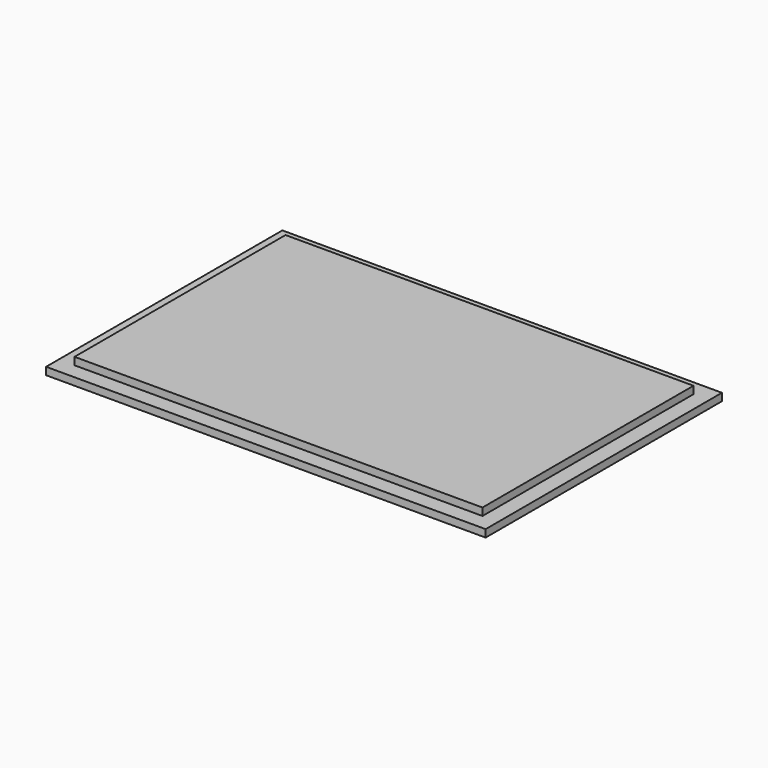
from build123d import *

# Parameters (mm, degrees)
F2_DEPTH = 105.9625
F3_W     = 176.60625
F3_H     = 3
F4_DEPTH = 6.35
F5_W     = 176.60625
F5_H     = 3
F6_DEPTH = 6.35


# Not quite as in the source:
# - a length typed as a fraction of an inch, garbled in the dataset ("3 / 203.2 mm" for 3/8 in), is restored


with BuildPart() as f2:
    # F1 (on Front) → F2 (new body)
    with BuildSketch(Plane.XZ):
        Polygon((-42.2606132925, -1.7798869123), (-42.2606132925, -4.7798869123), (134.3456367075, -4.7798869123), (134.3456367075, -1.7798869123), (127.9956367075, -1.7798869123), (127.9956367075, 1.2201130877), (-35.9106132925, 1.2201130877), (-35.9106132925, -1.7798869123), align=None)
    extrude(amount=F2_DEPTH)

    # F3 (on face) → F4 (join)
    with BuildSketch(Plane.XZ.offset(105.9625)):
        with Locations((46.0425117075, -3.2798869123)):
            Rectangle(F3_W, F3_H)
    extrude(amount=F4_DEPTH)

    # F5 (on face) → F6 (join)
    with BuildSketch(Plane(origin=(0, 0, 0), x_dir=(-1, 0, 0), z_dir=(0, 1, 0))):
        with Locations((-46.0425117075, -3.2798869123)):
            Rectangle(F5_W, F5_H)
    extrude(amount=F6_DEPTH)


solid = f2.part
